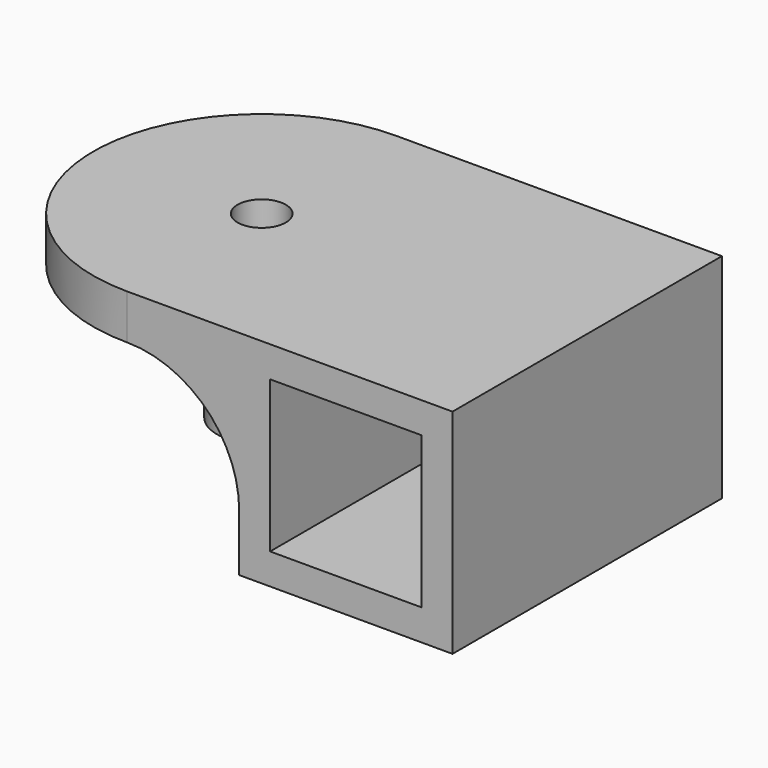
from build123d import *
from build123d import SkipClean  # not in build123d's __all__

# Parameters (mm, degrees)
F0_W         = 19
F0_H         = 19
F0_W_2       = 13.5
F0_H_2       = 13.5
F1_DEPTH     = 15
F2_R         = 4
F2_R_2       = 2.15
F3_DEPTH     = 4
F4_DEPTH     = 16
F5_T9_DEPTH  = 30
F5_S10_R     = 2.15
F5_T11_DEPTH = 18


# Not quite as in the source:
# - a fillet or chamfer that OpenCascade refuses, or shapes differently, is made with other operations: its cross-section is extruded or revolved along the edge and cut away or added


with BuildPart() as f1:
    # F0 (on Front) → F1 (new body, symmetric)
    with BuildSketch(Plane.XZ):
        Rectangle(F0_W, F0_H)
        Rectangle(F0_W_2, F0_H_2, mode=Mode.SUBTRACT)
    extrude(amount=F1_DEPTH, both=True)

    # F2 (on face) → F3 (join)
    with BuildSketch(Plane.XY.offset(9.5)):
        with BuildLine():
            Line((-9.5, -15), (-9.5, 15))
            Line((-9.5, 15), (-19.5, 15))
            ThreePointArc((-19.5, 15), (-34.5, 0), (-19.5, -15))
            Line((-19.5, -15), (-9.5, -15))
        make_face()
        with Locations((-19.5, 0)):
            Circle(F2_R, mode=Mode.SUBTRACT)
        with Locations((-19.5, 0)):
            Circle(F2_R)
        with Locations((-19.5, 0)):
            Circle(F2_R_2, mode=Mode.SUBTRACT)
    extrude(amount=-F3_DEPTH)

    # F2 (on face) → F4 (join)
    with BuildSketch(Plane.XY.offset(9.5)):
        with Locations((-19.5, 0)):
            Circle(F2_R)
        with Locations((-19.5, 0)):
            Circle(F2_R_2, mode=Mode.SUBTRACT)
    extrude(amount=-F4_DEPTH)

    # F5: fillet of radius 10 on 2 edges, made by hand


with BuildPart() as f5_tool2:
    # F5_s3 → F5_t4 (revolve)
    with BuildSketch(Plane.XZ):
        with BuildLine():
            ThreePointArc((-5.5, 5.5), (-12.5710678119, 2.5710678119), (-15.5, -4.5))
            Line((-15.5, -4.5), (-15.5, 5.5))
            Line((-15.5, 5.5), (-5.5, 5.5))
        make_face()
    revolve(axis=Axis((-19.5, 0, 5.5), (0, 0, 1)))

    split(bisect_by=Plane.YZ.offset(-6.75), keep=Keep.BOTTOM)


with BuildPart() as f1_1:
    add(f1.part, clean=False)

    # F5_t1: union F5_tool2
    add(f5_tool2.part)


with BuildPart() as f5_tool7:
    # F5_s8 → F5_t9 (new body)
    with BuildSketch(Plane.XZ.offset(15)):
        with BuildLine():
            ThreePointArc((-9.5, -4.5), (-12.4289321881, 2.5710678119), (-19.5, 5.5))
            Line((-19.5, 5.5), (-9.5, 5.5))
            Line((-9.5, 5.5), (-9.5, -4.5))
        make_face()
    extrude(amount=-F5_T9_DEPTH)

    # F5_s10 → F5_t11 (cut, symmetric)
    with BuildSketch(Plane.XY.offset(0.5)):
        with Locations((-19.5, 0)):
            Circle(F5_S10_R)
    with SkipClean():  # cleaning this boolean's faces spoils the solid; the shape is the same uncleaned
        extrude(amount=F5_T11_DEPTH, both=True, mode=Mode.SUBTRACT)


with BuildPart() as f1_2:
    add(f1_1.part, clean=False)

    # F5_t6: union F5_tool7
    add(f5_tool7.part)


solid = f1_2.part
